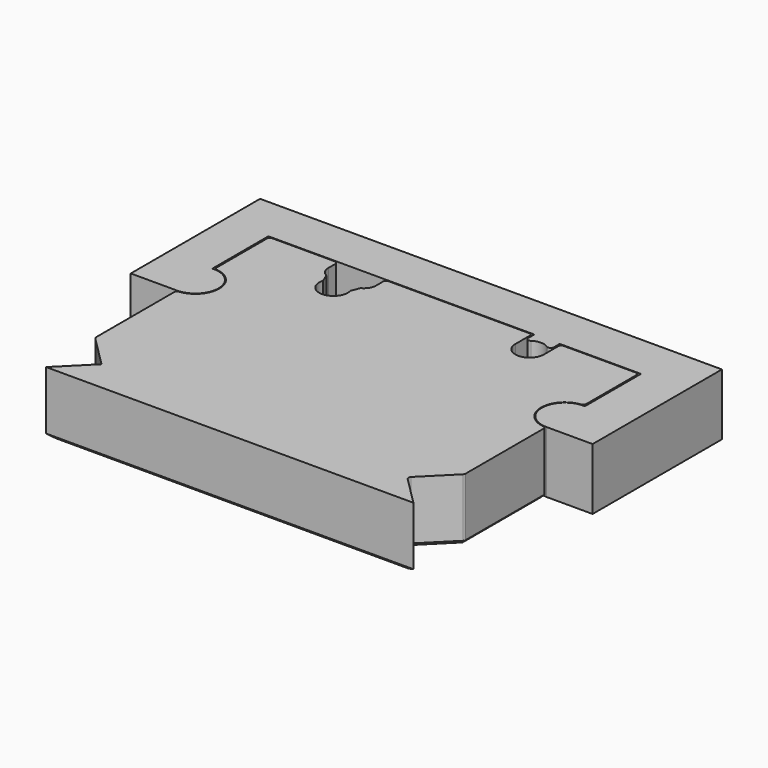
from build123d import *

# Parameters (mm, degrees)
F3_SIZE = 0.2
F6_R    = 0.2
F6_2_R  = 0.2


with BuildPart() as f2:
    # F2: sweep along a path in F1
    with BuildLine(Plane.XZ) as f2_path:
        Line((0, 0), (0, 4))
    # F0 (on Top) → F2 (sweep)
    with BuildSketch(Plane.XY):
        with BuildLine():
            Line((-9.9292893219, -13.925), (-11.9292893219, -15.925))
            Line((-11.9292893219, -15.925), (11.9292893219, -15.925))
            Line((11.9292893219, -15.925), (9.9292893219, -13.925))
            Line((9.9292893219, -13.925), (12, -11.8542893219))
            Line((12, -11.8542893219), (12, -5.2619319249))
            ThreePointArc((12, -5.2619319249), (10.45, -3.7119319249), (12, -2.1619319249))
            Line((12, -2.1619319249), (12, 2.2880680751))
            Line((12, 2.2880680751), (6.925, 2.2880680751))
            Line((6.925, 2.2880680751), (6.925, 0.925))
            ThreePointArc((6.925, 0.925), (6, 0), (5.075, 0.925))
            Line((5.075, 0.925), (5.075, 2.2880680751))
            Line((5.075, 2.2880680751), (-4.45, 2.2880680751))
            Line((-4.45, 2.2880680751), (-4.45, 1.5130680751))
            ThreePointArc((-4.45, 1.5130680751), (-4.5683478452, 1.1014457391), (-4.8872463162, 0.8155385424))
            Line((-4.8872463162, 0.8155385424), (-5.1123254204, 0.2601131305))
            ThreePointArc((-5.1123254204, 0.2601131305), (-6, -0.925), (-6.8876745796, 0.2601131305))
            Line((-6.8876745796, 0.2601131305), (-7.1127536838, 0.8155385424))
            ThreePointArc((-7.1127536838, 0.8155385424), (-7.4316521548, 1.1014457391), (-7.55, 1.5130680751))
            Line((-7.55, 1.5130680751), (-7.55, 2.2880680751))
            Line((-7.55, 2.2880680751), (-12, 2.2880680751))
            Line((-12, 2.2880680751), (-12, -2.1619319249))
            ThreePointArc((-12, -2.1619319249), (-10.45, -3.7119319249), (-12, -5.2619319249))
            Line((-12, -5.2619319249), (-12, -11.8542893219))
            Line((-12, -11.8542893219), (-9.9292893219, -13.925))
        make_face()
    sweep(path=f2_path.line)

    # F3
    f3_edges = [f2.edges().sort_by_distance(p)[0] for p in [
        (-10.929289, -14.925, 0),
        (0, -15.925, 0),
        (10.929289, -14.925, 0),
        (10.964645, -12.889645, 0),
        (12, -8.558111, 0),
        (10.45, -3.711932, 0),
        (12, 0.063068, 0),
        (9.4625, 2.288068, 0),
        (6.925, 1.606534, 0),
        (6, 0, 0),
        (5.075, 1.606534, 0),
        (0.3125, 2.288068, 0),
        (-4.45, 1.900568, 0),
        (-4.568348, 1.101446, 0),
        (-4.999786, 0.537826, 0),
        (-6, -0.925, 0),
        (-7.000214, 0.537826, 0),
        (-7.431652, 1.101446, 0),
        (-7.55, 1.900568, 0),
        (-9.775, 2.288068, 0),
        (-12, 0.063068, 0),
        (-10.45, -3.711932, 0),
        (-12, -8.558111, 0),
        (-10.964645, -12.889645, 0),
    ]]
    chamfer(f3_edges, length=F3_SIZE)

    # F6
    f6_edges = [f2.edges().sort_by_distance(p)[0] for p in [
        (-12, -11.854289, 2.1),
        (12, 2.288068, 2.1),
        (-7.55, 2.288068, 2.1),
        (-4.45, 2.288068, 2.1),
        (5.075, 2.288068, 2.1),
        (6.925, 2.288068, 2.1),
        (-12, -2.161932, 2.1),
        (12, -5.261932, 2.1),
        (-12, -5.261932, 2.1),
        (9.929289, -13.925, 2.1),
        (12, -11.854289, 2.1),
        (12, -2.161932, 2.1),
        (-12, 2.288068, 2.1),
    ]]
    fillet(f6_edges, radius=F6_R)


with BuildPart() as f5:
    # F5: sweep along a path in F1
    with BuildLine(Plane.XZ) as f5_path:
        Line((0, 0), (0, 4))
    # F4 (on Top) → F5 (sweep)
    with BuildSketch(Plane.XY):
        with BuildLine():
            ThreePointArc((-12, -5.2119319249), (-10.5, -3.7119319249), (-12, -2.2119319249))
            Line((-12, -2.2119319249), (-12.1, -2.2119319249))
            Line((-12.1, -2.2119319249), (-12.1, 2.3380680751))
            Line((-12.1, 2.3380680751), (0, 2.3380680751))
            Line((0, 2.3380680751), (5.175, 2.3380680751))
            Line((5.175, 2.3380680751), (6.825, 2.3380680751))
            Line((6.825, 2.3380680751), (12.1, 2.3380680751))
            Line((12.1, 2.3380680751), (12.1, -2.2119319249))
            Line((12.1, -2.2119319249), (12, -2.2119319249))
            ThreePointArc((12, -2.2119319249), (10.5, -3.7119319249), (12, -5.2119319249))
            Line((12, -5.2119319249), (15, -5.2119319249))
            Line((15, -5.2119319249), (15, 5.2880680751))
            Line((15, 5.2880680751), (0, 5.2880680751))
            Line((0, 5.2880680751), (-15, 5.2880680751))
            Line((-15, 5.2880680751), (-15, -5.2119319249))
            Line((-15, -5.2119319249), (-12, -5.2119319249))
        make_face()
        with BuildLine():
            Line((6.825, 2.3380680751), (5.175, 2.3380680751))
            Line((5.175, 2.3380680751), (5.175, 1.3433300133))
            ThreePointArc((5.175, 1.3433300133), (6, 1.85), (6.825, 1.3433300133))
            Line((6.825, 1.3433300133), (6.825, 2.3380680751))
        make_face()
    sweep(path=f5_path.line)

    # F6#2
    f6_2_edges = [f5.edges().sort_by_distance(p)[0] for p in [
        (5.175, 1.34333, 2),
        (6.825, 1.34333, 2),
    ]]
    fillet(f6_2_edges, radius=F6_2_R)


solid = Compound([f2.part, f5.part])
